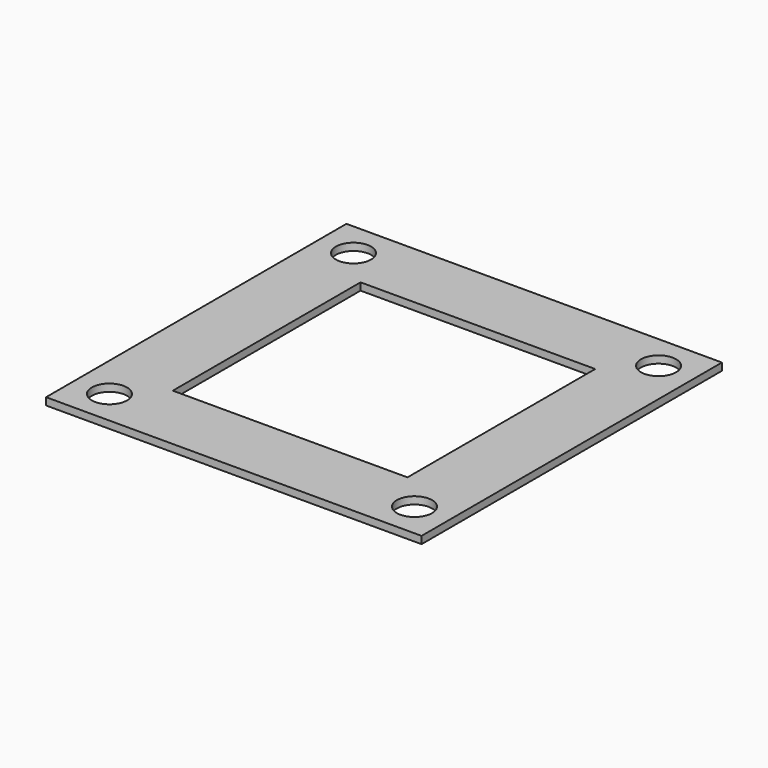
from build123d import *

# Parameters (mm, degrees)
F0_W     = 15.24
F0_H     = 15.24
F0_R     = 3.81
F0_W_2   = 50.8
F0_H_2   = 50.8
F1_DEPTH = 1.5875


# Not quite as in the source:
# - a feature names something its author has since deleted; it is built from what else it names


with BuildPart() as f1:
    # F0 (on Top) → F1 (new body)
    with BuildSketch(Plane.XY):
        with Locations((-39.3306643713, -48.6370485475)):
            Rectangle(F0_W, F0_H)
        with Locations((-39.3306643713, -48.6370485475)):
            Circle(F0_R, mode=Mode.SUBTRACT)
        with Locations((26.7093356287, -48.6370485475)):
            Rectangle(F0_W, F0_H)
        with Locations((26.7093356287, -48.6370485475)):
            Circle(F0_R, mode=Mode.SUBTRACT)
        with Locations((-39.3306643713, 17.4029514525)):
            Rectangle(F0_W, F0_H)
        with Locations((-39.3306643713, 17.4029514525)):
            Circle(F0_R, mode=Mode.SUBTRACT)
        with Locations((26.7093356287, 17.4029514525)):
            Rectangle(F0_W, F0_H)
        with Locations((26.7093356287, 17.4029514525)):
            Circle(F0_R, mode=Mode.SUBTRACT)
        with Locations((-6.3106643713, 17.4029514525)):
            Rectangle(F0_W_2, F0_H)
        with Locations((-6.3106643713, -48.6370485475)):
            Rectangle(F0_W_2, F0_H)
        with Locations((-39.3306643713, -15.6170485475)):
            Rectangle(F0_W, F0_H_2)
        with Locations((26.7093356287, -15.6170485475)):
            Rectangle(F0_W, F0_H_2)
    extrude(amount=F1_DEPTH)


solid = f1.part
